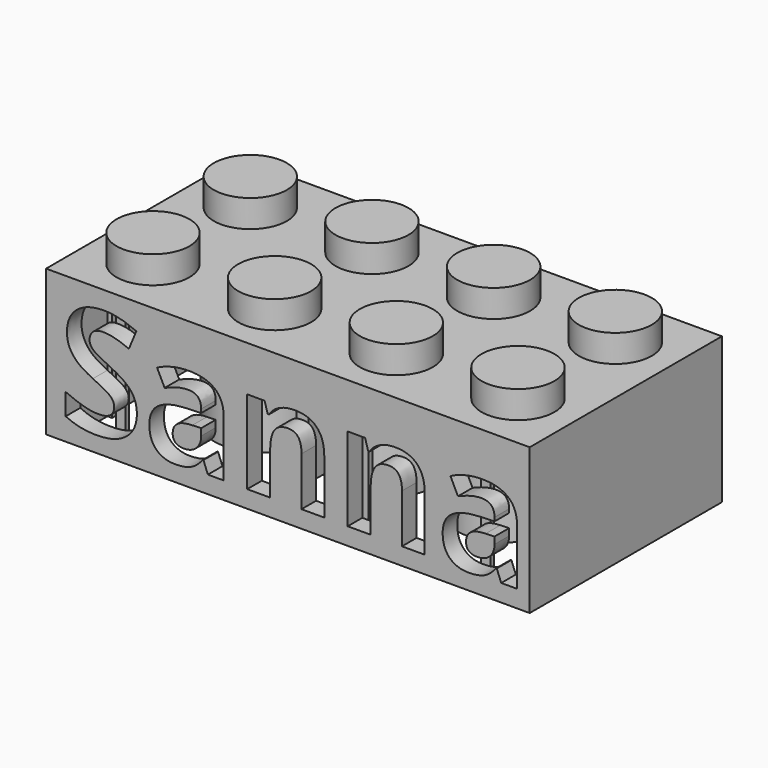
from build123d import *

# Parameters (mm, degrees)
F0_W          = 31.8
F0_H          = 15.8
F1_DEPTH      = 9.6
F2_W          = 29.4
F2_H          = 13.4
F3_DEPTH      = 8.4
F4_R          = 2.4
F5_DEPTH      = 1.8
F6_R          = 1.3
F7_DEPTH      = 1.2
F8_R          = 3.255
F8_R_2        = 2.4
F9_DEPTH      = 8.4
F10_W         = 0.6
F10_H         = 0.3
F11_DEPTH     = 8.4
F12_W         = 0.3
F12_H         = 0.6
F13_DEPTH     = 8.4
F14_W         = 0.8
F14_H         = 3.9
F14_H_2       = 3.8
F15_DEPTH     = 6.4
F16_TEXT_SIZE = 10.0543509082
F17_DEPTH     = 1.2


# Not quite as in the source:
# - Text() gives the source's letters only with a copy of the font that has no kerning and outlines rounded to 1/6400 em; it was checked with that copy


with BuildPart() as f1:
    # F0 (on Top) → F1 (new body)
    with BuildSketch(Plane.XY):
        Rectangle(F0_W, F0_H)
    extrude(amount=F1_DEPTH)

    # F2 (on face) → F3 (cut)
    with BuildSketch(Plane(origin=(0, 0, 0), x_dir=(1, 0, 0), z_dir=(0, 0, -1))):
        Rectangle(F2_W, F2_H)
    extrude(amount=-F3_DEPTH, mode=Mode.SUBTRACT)

    # F4 (on face) → F5 (join)
    with BuildSketch(Plane.XY.offset(9.6)):
        with Locations((-11.95, 3.95)):
            Circle(F4_R)
        with Locations((-11.95, -4.05)):
            Circle(F4_R)
        with Locations((-3.95, 3.95)):
            Circle(F4_R)
        with Locations((-3.95, -4.05)):
            Circle(F4_R)
        with Locations((4.05, 3.95)):
            Circle(F4_R)
        with Locations((4.05, -4.05)):
            Circle(F4_R)
        with Locations((12.05, 3.95)):
            Circle(F4_R)
        with Locations((12.05, -4.05)):
            Circle(F4_R)
    extrude(amount=F5_DEPTH)

    # F6 (on face) → F7 (cut)
    with BuildSketch(Plane(origin=(0, 0, 8.4), x_dir=(1, 0, 0), z_dir=(0, 0, -1))):
        with Locations((-11.95, 3.95)):
            Circle(F6_R)
        with Locations((-11.95, -4.05)):
            Circle(F6_R)
        with Locations((-3.95, 3.95)):
            Circle(F6_R)
        with Locations((-3.95, -4.05)):
            Circle(F6_R)
        with Locations((4.05, 3.95)):
            Circle(F6_R)
        with Locations((4.05, -4.05)):
            Circle(F6_R)
        with Locations((12.05, 3.95)):
            Circle(F6_R)
        with Locations((12.05, -4.05)):
            Circle(F6_R)
    extrude(amount=-F7_DEPTH, mode=Mode.SUBTRACT)

    # F8 (on face) → F9 (join, through all)
    with BuildSketch(Plane(origin=(0, 0, 8.4), x_dir=(1, 0, 0), z_dir=(0, 0, -1))):
        with Locations((-7.95, -0.05)):
            Circle(F8_R)
        with Locations((-7.95, -0.05)):
            Circle(F8_R_2, mode=Mode.SUBTRACT)
        with Locations((0.05, -0.05)):
            Circle(F8_R)
        with Locations((0.05, -0.05)):
            Circle(F8_R_2, mode=Mode.SUBTRACT)
        with Locations((8.05, -0.05)):
            Circle(F8_R)
        with Locations((8.05, -0.05)):
            Circle(F8_R_2, mode=Mode.SUBTRACT)
    extrude(amount=F9_DEPTH)

    # F10 (on face) → F11 (join, through all)
    with BuildSketch(Plane(origin=(0, 0, 0), x_dir=(1, 0, 0), z_dir=(0, 0, -1))):
        with Locations((-11.95, 6.55)):
            Rectangle(F10_W, F10_H)
        with Locations((-11.95, -6.55)):
            Rectangle(F10_W, F10_H)
        with Locations((-3.95, 6.55)):
            Rectangle(F10_W, F10_H)
        with Locations((-3.95, -6.55)):
            Rectangle(F10_W, F10_H)
        with Locations((4.05, 6.55)):
            Rectangle(F10_W, F10_H)
        with Locations((4.05, -6.55)):
            Rectangle(F10_W, F10_H)
        with Locations((12.05, 6.55)):
            Rectangle(F10_W, F10_H)
        with Locations((12.05, -6.55)):
            Rectangle(F10_W, F10_H)
    extrude(amount=-F11_DEPTH)

    # F12 (on Top) → F13 (join, through all)
    with BuildSketch(Plane.XY):
        with Locations((-14.55, -4.05)):
            Rectangle(F12_W, F12_H)
        with Locations((-14.55, 3.95)):
            Rectangle(F12_W, F12_H)
        with Locations((14.55, -4.05)):
            Rectangle(F12_W, F12_H)
        with Locations((14.55, 3.95)):
            Rectangle(F12_W, F12_H)
    extrude(amount=F13_DEPTH)

    # F14 (on face) → F15 (join)
    with BuildSketch(Plane(origin=(0, 0, 8.4), x_dir=(1, 0, 0), z_dir=(0, 0, -1))):
        with Locations((0, 4.95)):
            Rectangle(F14_W, F14_H)
        with Locations((0, -5)):
            Rectangle(F14_W, F14_H_2)
    extrude(amount=F15_DEPTH)

    # F16 (on face) → F17 (cut)
    with BuildSketch(Plane.XZ.offset(7.9)):
        with Locations((-15.0713149122, 1.1349548586)):
            Text('Sanna', F16_TEXT_SIZE, font='Open Sans', font_style=FontStyle.BOLD, text_align=(TextAlign.LEFT, TextAlign.BOTTOM))
    extrude(amount=-F17_DEPTH, mode=Mode.SUBTRACT)


solid = f1.part
